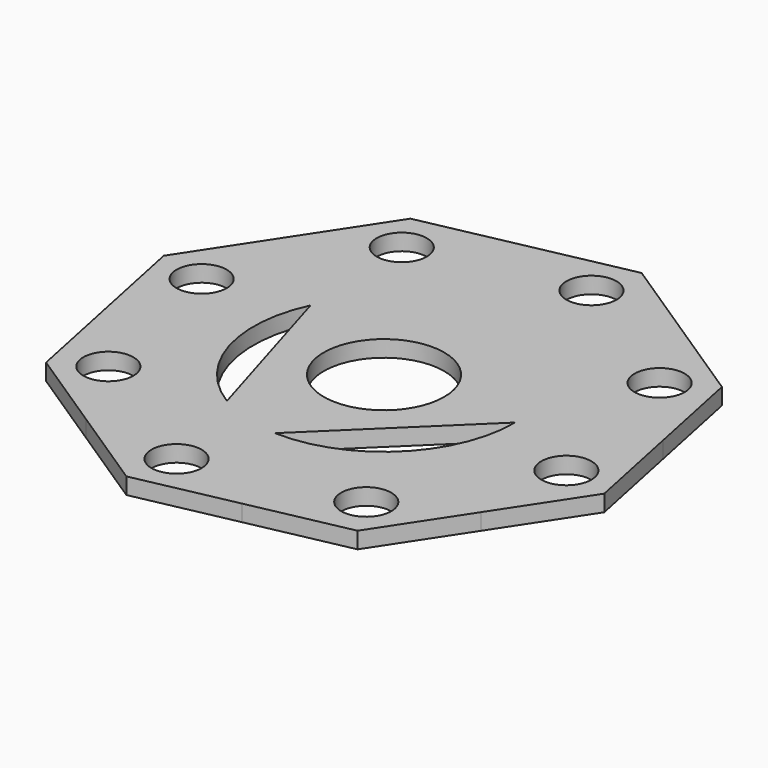
from build123d import *

# Parameters (mm, degrees)
F1_R     = 4.58
F1_R_2   = 11
F2_DEPTH = 3


# Not quite as in the source:
# - a feature names something its author has since deleted; it is built from what else it names


with BuildPart() as f2:
    # F1 (on face) → F2 (new body)
    with BuildSketch(Plane.XY):
        Polygon((24.5380218439, 37.3360185584), (9.072936592, 47.5), (-9.0495502624, 43.7515535479), (-27.1720371169, 40.0031070959), (-37.3360185584, 24.5380218439), (-47.5, 9.072936592), (-43.7515535479, -9.0495502624), (-40.0031070959, -27.1720371169), (-24.5380218439, -37.3360185584), (-9.072936592, -47.5), (9.0495502624, -43.7515535479), (27.1720371169, -40.0031070959), (37.3360185584, -24.5380218439), (47.5, -9.072936592), (43.7515535479, 9.0495502624), (40.0031070959, 27.1720371169), align=None)
        with Locations((-6.8599609456, -38.8043858107)):
            Circle(F1_R, mode=Mode.SUBTRACT)
        with Locations((-32.2895692498, -22.5881194432)):
            Circle(F1_R, mode=Mode.SUBTRACT)
        with BuildLine():
            ThreePointArc((-12.4312179995, -20.3423307182), (-22.8394812689, -6.8340101965), (-21.5614159426, 10.1710836469))
            Line((-21.5614159426, 10.1710836469), (-12.4312179995, -20.3423307182))
        make_face(mode=Mode.SUBTRACT)
        with Locations((22.5881194432, -32.2895692498)):
            Circle(F1_R, mode=Mode.SUBTRACT)
        with BuildLine():
            Line((-0.8588934675, -23.8245231224), (23.8395803729, 0.1414483779))
            ThreePointArc((23.8395803729, 0.1414483779), (16.601805328, -17.1092273306), (-0.8588934675, -23.8245231224))
        make_face(mode=Mode.SUBTRACT)
        with Locations((38.8043858107, -6.8599609456)):
            Circle(F1_R, mode=Mode.SUBTRACT)
        with Locations((-38.8043858107, 6.8599609456)):
            Circle(F1_R, mode=Mode.SUBTRACT)
        with Locations((-22.5881194432, 32.2895692498)):
            Circle(F1_R, mode=Mode.SUBTRACT)
        Circle(F1_R_2, mode=Mode.SUBTRACT)
        with BuildLine():
            ThreePointArc((-14.3344307522, 19.0491389572), (5.5013141945, 23.1965760864), (21.3620855471, 10.5833312845))
            Line((21.3620855471, 10.5833312845), (-14.3344307522, 19.0491389572))
        make_face(mode=Mode.SUBTRACT)
        with Locations((32.2895692498, 22.5881194432)):
            Circle(F1_R, mode=Mode.SUBTRACT)
        with Locations((6.8599609456, 38.8043858107)):
            Circle(F1_R, mode=Mode.SUBTRACT)
        with BuildLine():
            Line((-14.3344307522, 19.0491389572), (21.3620855471, 10.5833312845))
            ThreePointArc((21.3620855471, 10.5833312845), (5.5013141945, 23.1965760864), (-14.3344307522, 19.0491389572))
        make_face()
    extrude(amount=F2_DEPTH)


solid = f2.part
